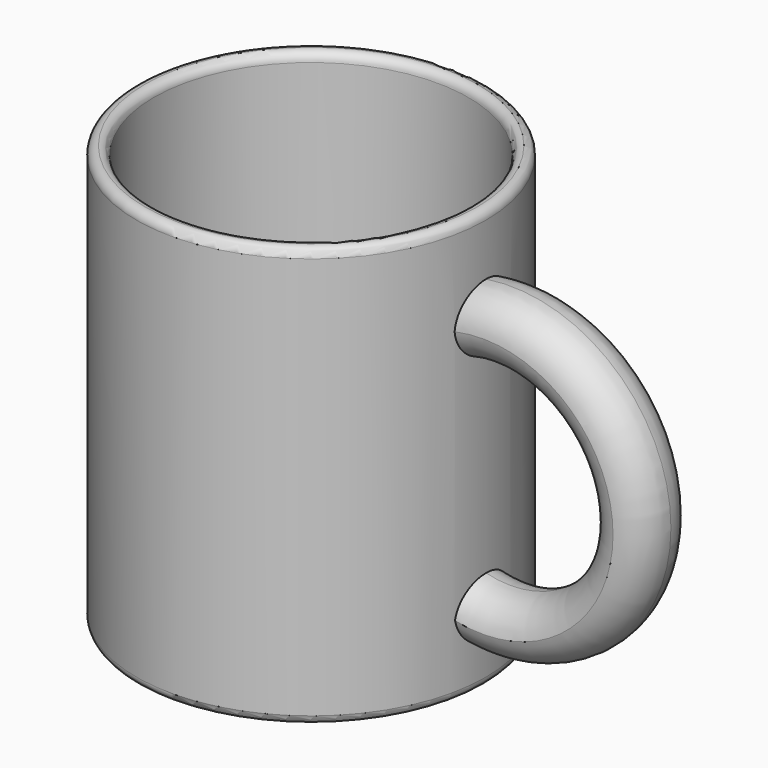
from build123d import *

# Parameters (mm, degrees)
F0_R         = 63.5
F2_DEPTH     = 152.4
F3_T         = -6.35
F4_DEPTH     = 12.7
F5_DEPTH     = 152.4
F6_T4_ANGLE  = 262.3827679328
F6_S5_R      = 63.5
F6_T6_DEPTH  = 84
F6_T10_ANGLE = 262.3827679328
F6_S11_R     = 63.5
F6_T12_DEPTH = 84
F6_T16_ANGLE = 313.645065155
F6_S17_R     = 63.5
F6_T18_DEPTH = 84
F6_T22_ANGLE = 313.645065155
F6_S23_R     = 63.5
F6_T24_DEPTH = 84
F7_R         = 3.17499


# Not quite as in the source:
# - a fillet or chamfer that OpenCascade refuses, or shapes differently, is made with other operations: its cross-section is extruded or revolved along the edge and cut away or added
# - a fillet or chamfer is up to 0.001 mm smaller than in the source, because OpenCascade refuses the exact size


with BuildPart() as f2:
    # F0 (on Top) → F2 (new body)
    with BuildSketch(Plane.XY):
        Circle(F0_R)
    extrude(amount=F2_DEPTH)

    # F3
    f3_openings = [f2.faces().sort_by_distance(p)[0] for p in [
        (0, 0, 152.4),
    ]]
    offset(amount=F3_T, openings=f3_openings)

    # F1 (on Front) → F4 (join, symmetric)
    with BuildSketch(Plane.XZ):
        with BuildLine():
            Line((49.501311034, 43.5545518994), (49.501311034, 19.0017146287))
            ThreePointArc((49.501311034, 19.0017146287), (130.6394136759, 72.7063623934), (49.5013073087, 126.4110045299))
            Line((49.5013073087, 126.4110045299), (49.5013073087, 99.5260253549))
            ThreePointArc((49.5013073087, 99.5260253549), (108.7160258507, 71.5402925683), (49.501311034, 43.5545518994))
        make_face()
    extrude(amount=F4_DEPTH, both=True)

    # F5 (cut): a face of the model
    f5_faces = [f2.faces().sort_by_distance(p)[0] for p in [
        (0, 0, 6.35),
    ]]
    extrude(f5_faces, amount=F5_DEPTH, mode=Mode.SUBTRACT)

    # F6: fillet of radius 12.7 on 4 edges, made by hand


with BuildPart() as f6_tool2:
    # F6_s3 → F6_t4 (revolve)
    with BuildSketch(Plane(origin=(4.9077736373, 0, -4.2951275785), x_dir=(0, 1, 0), z_dir=(-0.7525139529, 0, 0.6585763059))):
        with BuildLine():
            ThreePointArc((-12.7, -56.6832774583), (-8.9802561211, -47.7030213372), (0, -43.9832774583))
            Line((0, -43.9832774583), (0, -43.7292774583))
            Line((0, -43.7292774583), (-12.954, -43.7292774583))
            Line((-12.954, -43.7292774583), (-12.954, -56.6832774583))
            Line((-12.954, -56.6832774583), (-12.7, -56.6832774583))
        make_face()
    revolve(axis=Axis((72.2970297265, -12.7, 72.7063603699), (0, -1, 0)), revolution_arc=F6_T4_ANGLE)

    # F6_s5 → F6_t6 (cut, symmetric)
    with BuildSketch(Plane.XY.offset(72.7)):
        Circle(F6_S5_R)
    extrude(amount=F6_T6_DEPTH, both=True, mode=Mode.SUBTRACT)


with BuildPart() as f2_1:
    add(f2.part)

    # F6_t1: cut F6_tool2
    add(f6_tool2.part, mode=Mode.SUBTRACT)


with BuildPart() as f6_tool8:
    # F6_s9 → F6_t10 (revolve)
    with BuildSketch(Plane(origin=(4.9077736373, 0, -4.2951275785), x_dir=(0, 1, 0), z_dir=(-0.7525139529, 0, 0.6585763059))):
        with BuildLine():
            ThreePointArc((12.7, -56.6832774583), (8.9802561211, -47.7030213372), (0, -43.9832774583))
            Line((0, -43.9832774583), (0, -43.7292774583))
            Line((0, -43.7292774583), (12.954, -43.7292774583))
            Line((12.954, -43.7292774583), (12.954, -56.6832774583))
            Line((12.954, -56.6832774583), (12.7, -56.6832774583))
        make_face()
    revolve(axis=Axis((72.2970297265, 12.7, 72.7063603699), (0, -1, 0)), revolution_arc=F6_T10_ANGLE)

    # F6_s11 → F6_t12 (cut, symmetric)
    with BuildSketch(Plane.XY.offset(72.7)):
        Circle(F6_S11_R)
    extrude(amount=F6_T12_DEPTH, both=True, mode=Mode.SUBTRACT)


with BuildPart() as f2_2:
    add(f2_1.part)

    # F6_t7: cut F6_tool8
    add(f6_tool8.part, mode=Mode.SUBTRACT)


with BuildPart() as f6_tool14:
    # F6_s15 → F6_t16 (revolve)
    with BuildSketch(Plane(origin=(37.1142669501, 0, 86.6882103357), x_dir=(0, 1, 0), z_dir=(-0.3935804129, 0, -0.9192901928))):
        with BuildLine():
            ThreePointArc((0, 2.2668933091), (-8.9802561211, -1.4528505698), (-12.7, -10.4331066909))
            Line((-12.7, -10.4331066909), (-12.954, -10.4331066909))
            Line((-12.954, -10.4331066909), (-12.954, 2.5208933091))
            Line((-12.954, 2.5208933091), (0, 2.5208933091))
            Line((0, 2.5208933091), (0, 2.2668933091))
        make_face()
    revolve(axis=Axis((72.495434314, -12.7, 71.5402901576), (0, 1, 0)), revolution_arc=F6_T16_ANGLE)

    # F6_s17 → F6_t18 (cut, symmetric)
    with BuildSketch(Plane.XY.offset(71.5)):
        Circle(F6_S17_R)
    extrude(amount=F6_T18_DEPTH, both=True, mode=Mode.SUBTRACT)


with BuildPart() as f2_3:
    add(f2_2.part)

    # F6_t13: cut F6_tool14
    add(f6_tool14.part, mode=Mode.SUBTRACT)


with BuildPart() as f6_tool20:
    # F6_s21 → F6_t22 (revolve)
    with BuildSketch(Plane(origin=(37.1142669501, 0, 86.6882103357), x_dir=(0, 1, 0), z_dir=(-0.3935804129, 0, -0.9192901928))):
        with BuildLine():
            ThreePointArc((12.7, -10.4331066909), (8.9802561211, -1.4528505698), (0, 2.2668933091))
            Line((0, 2.2668933091), (0, 2.5208933091))
            Line((0, 2.5208933091), (12.954, 2.5208933091))
            Line((12.954, 2.5208933091), (12.954, -10.4331066909))
            Line((12.954, -10.4331066909), (12.7, -10.4331066909))
        make_face()
    revolve(axis=Axis((72.495434314, 12.7, 71.5402901576), (0, 1, 0)), revolution_arc=F6_T22_ANGLE)

    # F6_s23 → F6_t24 (cut, symmetric)
    with BuildSketch(Plane.XY.offset(71.5)):
        Circle(F6_S23_R)
    extrude(amount=F6_T24_DEPTH, both=True, mode=Mode.SUBTRACT)


with BuildPart() as f2_4:
    add(f2_3.part)

    # F6_t19: cut F6_tool20
    add(f6_tool20.part, mode=Mode.SUBTRACT)

    # F7 (radius 3.175 in the source; OpenCascade refuses exactly that, so slightly less here)
    f7_edges = [f2_4.edges().sort_by_distance(p)[0] for p in [
        (-63.5, 0, 152.4),
        (-57.15, 0, 152.4),
        (-63.5, 0, 0),
    ]]
    fillet(f7_edges, radius=F7_R)


solid = f2_4.part
